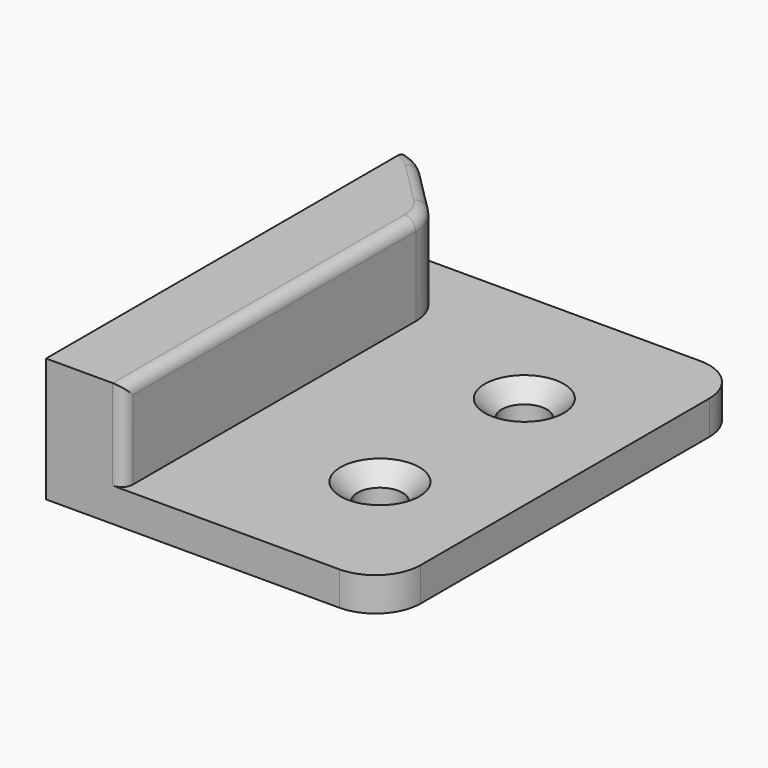
from build123d import *

# Parameters (mm, degrees)
F0_W        = 6.9
F0_H        = 40
F1_DEPTH    = 11
F0_W_2      = 23.1
F0_R        = 2
F2_DEPTH    = 3
F3_SIZE     = 6
F4_T1_DEPTH = 11.8208999069
F4_T3_DEPTH = 12.1421356237
F4_T5_DEPTH = 23
F5_SIZE     = 1.5
F6_R        = 1


# Not quite as in the source:
# - a fillet or chamfer that OpenCascade refuses, or shapes differently, is made with other operations: its cross-section is extruded or revolved along the edge and cut away or added


with BuildPart() as f1:
    # F0 (on Top) → F1 (new body)
    with BuildSketch(Plane.XY):
        with Locations((3.45, 20)):
            Rectangle(F0_W, F0_H)
    extrude(amount=F1_DEPTH)

    # F0 (on Top) → F2 (join)
    with BuildSketch(Plane.XY):
        with Locations((18.45, 20)):
            Rectangle(F0_W_2, F0_H)
        with Locations((20, 12)):
            Circle(F0_R, mode=Mode.SUBTRACT)
        with Locations((20, 28)):
            Circle(F0_R, mode=Mode.SUBTRACT)
    extrude(amount=F2_DEPTH)

    # F3
    f3_edges = [f1.edges().sort_by_distance(p)[0] for p in [
        (6.9, 40, 7),
    ]]
    chamfer(f3_edges, length=F3_SIZE)

    # F4: fillet of radius 4 on 4 edges, made by hand

    # F4_s2 → F4_t1 (cut)
    with BuildSketch(Plane.XY.offset(3)):
        with BuildLine():
            ThreePointArc((0, 40), (1.0681383035, 39.602199685), (1.9807136938, 38.9192863062))
            Line((1.9807136938, 38.9192863062), (0.9, 40))
            Line((0.9, 40), (0, 40))
        make_face()
    extrude(amount=F4_T1_DEPTH, mode=Mode.SUBTRACT)

    # F4_s4 → F4_t3 (cut)
    with BuildSketch(Plane.XY.offset(3)):
        with BuildLine():
            ThreePointArc((5.7284271247, 35.1715728753), (6.59551813, 33.87387948), (6.9, 32.3431457505))
            Line((6.9, 32.3431457505), (6.9, 34))
            Line((6.9, 34), (5.7284271247, 35.1715728753))
        make_face()
    extrude(amount=F4_T3_DEPTH, mode=Mode.SUBTRACT)

    # F4_s6 → F4_t5 (cut)
    with BuildSketch(Plane.XY.offset(-10)):
        with BuildLine():
            ThreePointArc((26, 40), (28.8284271247, 38.8284271247), (30, 36))
            Line((30, 36), (30, 40))
            Line((30, 40), (26, 40))
        make_face()
        with BuildLine():
            ThreePointArc((30, 4), (28.8284271247, 1.1715728753), (26, 0))
            Line((26, 0), (30, 0))
            Line((30, 0), (30, 4))
        make_face()
    extrude(amount=F4_T5_DEPTH, mode=Mode.SUBTRACT)

    # F5
    f5_edges = [f1.edges().sort_by_distance(p)[0] for p in [
        (18, 28, 3),
        (18, 12, 3),
    ]]
    chamfer(f5_edges, length=F5_SIZE)

    # F6
    f6_edges = [f1.edges().sort_by_distance(p)[0] for p in [
        (6.9, 0, 7),
        (6.9, 16.171573, 11),
        (6.595518, 33.873879, 11),
        (3.85457, 37.04543, 11),
        (1.068138, 39.6022, 11),
    ]]
    fillet(f6_edges, radius=F6_R)


solid = f1.part
